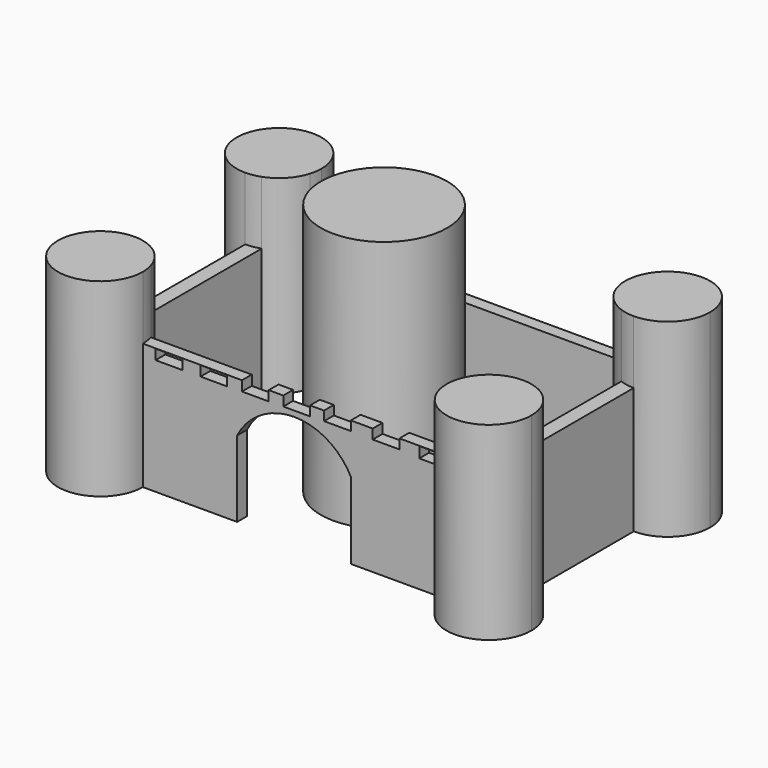
from build123d import *

# Parameters (mm, degrees)
F1_DEPTH = 25.4
F2_DEPTH = 38.1
F0_R     = 12.7
F3_DEPTH = 50.8
F4_W     = 5.3753480315
F4_H     = 2.0379073262
F4_H_2   = 2.001611045
F4_H_3   = 1.9500455767
F4_H_4   = 1.8769497931
F4_H_5   = 2.1840970308
F4_H_6   = 2.4033825189
F5_DEPTH = 25.4


with BuildPart() as f1:
    # F0 (on Top) → F1 (new body)
    with BuildSketch(Plane.XY):
        with BuildLine():
            ThreePointArc((30.9043610914, 19.9963377189), (30.6327265804, 21.213579998), (30.5415316269, 22.4574238604))
            Line((30.5415316269, 22.4574238604), (-30.5415316269, 22.4574238604))
            ThreePointArc((-30.5415316269, 22.4574238604), (-30.6327265804, 21.213579998), (-30.9043610914, 19.9963377189))
            Line((-30.9043610914, 19.9963377189), (30.9043610914, 19.9963377189))
        make_face()
    extrude(amount=F1_DEPTH)


with BuildPart() as f1b:
    # F0 (on Top) → F1, piece 2 (new body)
    with BuildSketch(Plane.XY):
        with BuildLine():
            ThreePointArc((-36.1472253967, 14.4455857303), (-37.585860411, 14.059279949), (-39.0697670953, 13.929188392))
            Line((-39.0697670953, 13.929188392), (-39.0697670953, -13.929188392))
            ThreePointArc((-39.0697670953, -13.929188392), (-37.585860411, -14.059279949), (-36.1472253967, -14.4455857303))
            Line((-36.1472253967, -14.4455857303), (-36.1472253967, 14.4455857303))
        make_face()
    extrude(amount=F1_DEPTH)


with BuildPart() as f1c:
    # F0 (on Top) → F1, piece 3 (new body)
    with BuildSketch(Plane.XY):
        with BuildLine():
            ThreePointArc((-30.9043610914, -19.9963377189), (-30.6327265804, -21.213579998), (-30.5415316269, -22.4574238604))
            Line((-30.5415316269, -22.4574238604), (30.5415316269, -22.4574238604))
            ThreePointArc((30.5415316269, -22.4574238604), (30.6327265804, -21.213579998), (30.9043610914, -19.9963377189))
            Line((30.9043610914, -19.9963377189), (-30.9043610914, -19.9963377189))
        make_face()
    extrude(amount=F1_DEPTH)

    # F4 (on face) → F5 (cut)
    with BuildSketch(Plane.XZ.offset(22.4574238604)):
        with BuildLine():
            Line((-11.5776741877, 15.2990696952), (-11.5776741877, 0))
            Line((-11.5776741877, 0), (11.3709308207, 0))
            Line((11.3709308207, 0), (11.3709308207, 15.2990696952))
            ThreePointArc((11.3709308207, 15.2990696952), (-0.1033716835, 22.3287878897), (-11.5776741877, 15.2990696952))
        make_face()
        with Locations((-34.3195348978, 24.3810463369)):
            Rectangle(F4_W, F4_H)
        with Locations((-25.2913832664, 24.3237949908)):
            Rectangle(F4_W, F4_H)
        with Locations((-16.2510816008, 24.3512634188)):
            Rectangle(F4_W, F4_H)
        with Locations((-7.9092020169, 24.3991944775)):
            Rectangle(F4_W, F4_H_2)
        with Locations((0.400578283, 24.4249772117)):
            Rectangle(F4_W, F4_H_3)
        with Locations((8.5872309282, 24.4615251034)):
            Rectangle(F4_W, F4_H_4)
        with Locations((18.3819765225, 24.4249772117)):
            Rectangle(F4_W, F4_H_3)
        with Locations((27.7381502092, 24.249621667)):
            Rectangle(F4_W, F4_H_5)
        with Locations((37.9714630544, 24.3592662737)):
            Rectangle(F4_W, F4_H_6)
    extrude(amount=-F5_DEPTH, mode=Mode.SUBTRACT)


with BuildPart() as f1d:
    # F0 (on Top) → F1, piece 4 (new body)
    with BuildSketch(Plane.XY):
        with BuildLine():
            Line((39.0697670953, -13.929188392), (39.0697670953, 13.929188392))
            ThreePointArc((39.0697670953, 13.929188392), (37.585860411, 14.059279949), (36.1472253967, 14.4455857303))
            Line((36.1472253967, 14.4455857303), (36.1472253967, -14.4455857303))
            ThreePointArc((36.1472253967, -14.4455857303), (37.585860411, -14.059279949), (39.0697670953, -13.929188392))
        make_face()
    extrude(amount=F1_DEPTH)


with BuildPart() as f2:
    # F0 (on Top) → F2 (new body)
    with BuildSketch(Plane.XY):
        with BuildLine():
            ThreePointArc((47.5980025637, 22.4574238604), (39.0697670953, 30.9856593288), (30.5415316269, 22.4574238604))
            ThreePointArc((30.5415316269, 22.4574238604), (30.6327265804, 21.213579998), (30.9043610914, 19.9963377189))
            ThreePointArc((30.9043610914, 19.9963377189), (32.8698995183, 16.6014489432), (36.1472253967, 14.4455857303))
            ThreePointArc((36.1472253967, 14.4455857303), (37.585860411, 14.059279949), (39.0697670953, 13.929188392))
            ThreePointArc((39.0697670953, 13.929188392), (45.1001402266, 16.4270507292), (47.5980025637, 22.4574238604))
        make_face()
    extrude(amount=F2_DEPTH)


with BuildPart() as f2b:
    # F0 (on Top) → F2, piece 2 (new body)
    with BuildSketch(Plane.XY):
        with BuildLine():
            ThreePointArc((47.5980025637, -22.4574238604), (45.1001402266, -16.4270507292), (39.0697670953, -13.929188392))
            ThreePointArc((39.0697670953, -13.929188392), (37.585860411, -14.059279949), (36.1472253967, -14.4455857303))
            ThreePointArc((36.1472253967, -14.4455857303), (32.8698995183, -16.6014489432), (30.9043610914, -19.9963377189))
            ThreePointArc((30.9043610914, -19.9963377189), (30.6327265804, -21.213579998), (30.5415316269, -22.4574238604))
            ThreePointArc((30.5415316269, -22.4574238604), (39.0697670953, -30.9856593288), (47.5980025637, -22.4574238604))
        make_face()
    extrude(amount=F2_DEPTH)


with BuildPart() as f2c:
    # F0 (on Top) → F2, piece 3 (new body)
    with BuildSketch(Plane.XY):
        with BuildLine():
            ThreePointArc((-36.1472253967, -14.4455857303), (-37.585860411, -14.059279949), (-39.0697670953, -13.929188392))
            ThreePointArc((-39.0697670953, -13.929188392), (-45.1001402266, -28.4877969917), (-30.5415316269, -22.4574238604))
            ThreePointArc((-30.5415316269, -22.4574238604), (-30.6327265804, -21.213579998), (-30.9043610914, -19.9963377189))
            ThreePointArc((-30.9043610914, -19.9963377189), (-32.8698995183, -16.6014489432), (-36.1472253967, -14.4455857303))
        make_face()
    extrude(amount=F2_DEPTH)


with BuildPart() as f2d:
    # F0 (on Top) → F2, piece 4 (new body)
    with BuildSketch(Plane.XY):
        with BuildLine():
            ThreePointArc((-30.9043610914, 19.9963377189), (-30.6327265804, 21.213579998), (-30.5415316269, 22.4574238604))
            ThreePointArc((-30.5415316269, 22.4574238604), (-45.1001402266, 28.4877969917), (-39.0697670953, 13.929188392))
            ThreePointArc((-39.0697670953, 13.929188392), (-37.585860411, 14.059279949), (-36.1472253967, 14.4455857303))
            ThreePointArc((-36.1472253967, 14.4455857303), (-32.8698995183, 16.6014489432), (-30.9043610914, 19.9963377189))
        make_face()
    extrude(amount=F2_DEPTH)


with BuildPart() as f3:
    # F0 (on Top) → F3 (new body)
    with BuildSketch(Plane.XY):
        Circle(F0_R)
    extrude(amount=F3_DEPTH)


solid = Compound([f1.part, f1b.part, f1c.part, f1d.part, f2.part, f2b.part, f2c.part, f2d.part, f3.part])
